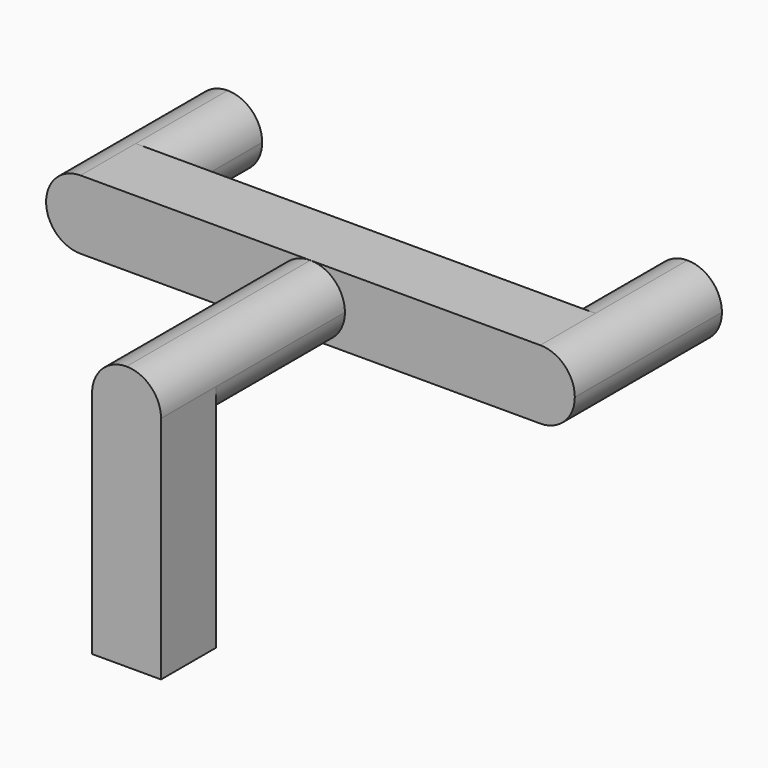
from build123d import *

# Parameters (mm, degrees)
F1_DEPTH  = 50
F2_DEPTH  = 50
F3_DEPTH  = 30
F5_DEPTH  = 100
F8_R      = 15
F9_DEPTH  = 50
F10_W     = 15
F10_H     = 30
F11_DEPTH = 100


with BuildPart() as f1:
    # F0 (on Front) → F1 (new body)
    with BuildSketch(Plane.XZ):
        with BuildLine():
            Line((-100, -15), (-100, 15))
            ThreePointArc((-100, 15), (-115, 0), (-100, -15))
        make_face()
        with BuildLine():
            ThreePointArc((-100, -15), (-89.393398, -10.606602), (-85, 0))
            ThreePointArc((-85, 0), (-89.393398, 10.606602), (-100, 15))
            Line((-100, 15), (-100, -15))
        make_face()
    extrude(amount=-F1_DEPTH)



with BuildPart() as f1b:
    # F0 (on Front) → F1, piece 2 (new body)
    with BuildSketch(Plane.XZ):
        with BuildLine():
            Line((100, -15), (100, 15))
            ThreePointArc((100, 15), (85, 0), (100, -15))
        make_face()
        with BuildLine():
            ThreePointArc((115, 0), (110.606602, 10.606602), (100, 15))
            Line((100, 15), (100, -15))
            ThreePointArc((100, -15), (110.606602, -10.606602), (115, 0))
        make_face()
    extrude(amount=-F1_DEPTH)


with BuildPart() as f2:
    # F0 (on Front) → F2 (new body)
    with BuildSketch(Plane.XZ):
        with BuildLine():
            Line((-100, -15), (-100, 15))
            ThreePointArc((-100, 15), (-115, 0), (-100, -15))
        make_face()
        with BuildLine():
            ThreePointArc((-100, -15), (-89.393398, -10.606602), (-85, 0))
            ThreePointArc((-85, 0), (-89.393398, 10.606602), (-100, 15))
            Line((-100, 15), (-100, -15))
        make_face()
    extrude(amount=-F2_DEPTH)


with BuildPart() as f2b:
    # F0 (on Front) → F2, piece 2 (new body)
    with BuildSketch(Plane.XZ):
        with BuildLine():
            Line((100, -15), (100, 15))
            ThreePointArc((100, 15), (85, 0), (100, -15))
        make_face()
        with BuildLine():
            ThreePointArc((115, 0), (110.606602, 10.606602), (100, 15))
            Line((100, 15), (100, -15))
            ThreePointArc((100, -15), (110.606602, -10.606602), (115, 0))
        make_face()
    extrude(amount=-F2_DEPTH)


with BuildPart() as f3:
    # F0 (on Front) → F3 (new body)
    with BuildSketch(Plane.XZ):
        with BuildLine():
            ThreePointArc((-100, 15), (-89.393398, 10.606602), (-85, 0))
            ThreePointArc((-85, 0), (-89.393398, -10.606602), (-100, -15))
            Line((-100, -15), (100, -15))
            ThreePointArc((100, -15), (85, 0), (100, 15))
            Line((100, 15), (-100, 15))
        make_face()
        with BuildLine():
            Line((-100, -15), (-100, 15))
            ThreePointArc((-100, 15), (-115, 0), (-100, -15))
        make_face()
        with BuildLine():
            ThreePointArc((-100, -15), (-89.393398, -10.606602), (-85, 0))
            ThreePointArc((-85, 0), (-89.393398, 10.606602), (-100, 15))
            Line((-100, 15), (-100, -15))
        make_face()
        with BuildLine():
            Line((100, -15), (100, 15))
            ThreePointArc((100, 15), (85, 0), (100, -15))
        make_face()
        with BuildLine():
            ThreePointArc((115, 0), (110.606602, 10.606602), (100, 15))
            Line((100, 15), (100, -15))
            ThreePointArc((100, -15), (110.606602, -10.606602), (115, 0))
        make_face()
    extrude(amount=F3_DEPTH)

    # F4 (on face) → F5 (join)
    with BuildSketch(Plane.XZ.offset(30)):
        with BuildLine():
            ThreePointArc((0, -15), (10.606602, -10.606602), (15, 0))
            ThreePointArc((15, 0), (10.606602, 10.606602), (0, 15))
            ThreePointArc((0, 15), (-15, 0), (0, -15))
        make_face()
    extrude(amount=F5_DEPTH)


with BuildPart() as f1_1:
    add(f1.part)

    add(f1b.part)  # F9 merges F1b

    add(f3.part)  # F9 merges F3
    # F8 (on face) → F9 (join)
    with BuildSketch(Plane(origin=(0, 0, 0), x_dir=(-1, 0, 0), z_dir=(0, 1, 0))):
        with Locations((100, 0)):
            Circle(F8_R)
        with Locations((-100, 0)):
            Circle(F8_R)
    extrude(amount=F9_DEPTH)

    # F10 (on Top) → F11 (join)
    with BuildSketch(Plane.XY):
        with Locations((7.5, -115)):
            Rectangle(F10_W, F10_H)
        with Locations((-7.5, -115)):
            Rectangle(F10_W, F10_H)
    extrude(amount=-F11_DEPTH)


solid = f1_1.part
